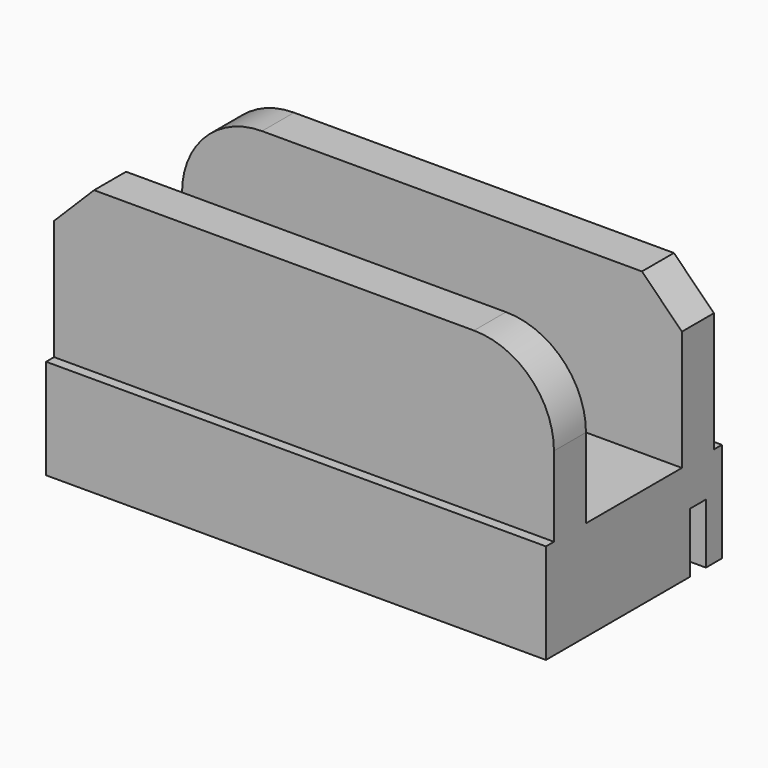
from build123d import *

# Parameters (mm, degrees)
F0_W      = 125
F0_H      = 25
F1_DEPTH  = 55
F2_W      = 125
F2_H      = 40
F3_DEPTH  = 52.5
F4_W      = 125
F4_H      = 40
F5_DEPTH  = 2.5
F6_W      = 30
F6_H      = 40
F7_DEPTH  = 125.001
F8_SIZE   = 10
F9_R      = 20
F10_SIZE  = 10
F11_R     = 20
F12_W     = 5
F12_H     = 15
F13_DEPTH = 125.001
F15_DEPTH = 25.001


with BuildPart() as f1:
    # F0 (on Front) → F1 (new body)
    with BuildSketch(Plane.XZ):
        Rectangle(F0_W, F0_H)
    extrude(amount=F1_DEPTH)

    # F2 (on face) → F3 (join)
    with BuildSketch(Plane.XZ.offset(55)):
        with Locations((0, 32.5)):
            Rectangle(F2_W, F2_H)
    extrude(amount=-F3_DEPTH)

    # F4 (on face) → F5 (cut)
    with BuildSketch(Plane.XZ.offset(55)):
        with Locations((0, 32.5)):
            Rectangle(F4_W, F4_H)
    extrude(amount=-F5_DEPTH, mode=Mode.SUBTRACT)

    # F6 (on face) → F7 (cut, through all)
    with BuildSketch(Plane(origin=(-62.5, 0, 0), x_dir=(0, -1, 0), z_dir=(-1, 0, 0))):
        with Locations((27.5, 32.5)):
            Rectangle(F6_W, F6_H)
    extrude(amount=-F7_DEPTH, mode=Mode.SUBTRACT)

    # F8
    f8_edges = [f1.edges().sort_by_distance(p)[0] for p in [
        (-62.5, -47.5, 52.5),
    ]]
    chamfer(f8_edges, length=F8_SIZE)

    # F9
    f9_edges = [f1.edges().sort_by_distance(p)[0] for p in [
        (-62.5, -7.5, 52.5),
    ]]
    fillet(f9_edges, radius=F9_R)

    # F10
    f10_edges = [f1.edges().sort_by_distance(p)[0] for p in [
        (62.5, -7.5, 52.5),
    ]]
    chamfer(f10_edges, length=F10_SIZE)

    # F11
    f11_edges = [f1.edges().sort_by_distance(p)[0] for p in [
        (62.5, -47.5, 52.5),
    ]]
    fillet(f11_edges, radius=F11_R)

    # F12 (on face) → F13 (cut, through all)
    with BuildSketch(Plane(origin=(-62.5, 0, 0), x_dir=(0, -1, 0), z_dir=(-1, 0, 0))):
        with Locations((7.5, -5)):
            Rectangle(F12_W, F12_H)
    extrude(amount=-F13_DEPTH, mode=Mode.SUBTRACT)

    # F14 (on face) → F15 (cut, through all)
    with BuildSketch(Plane.XY.offset(12.5)):
        with BuildLine():
            ThreePointArc((7e-10, -42.5), (10.606601718, -38.1066017176), (15, -27.5))
            ThreePointArc((15, -27.5), (10.6066017178, -16.8933982822), (0, -12.5))
            ThreePointArc((0, -12.5), (-15, -27.5000000003), (7e-10, -42.5))
        make_face()
    extrude(amount=-F15_DEPTH, mode=Mode.SUBTRACT)


solid = f1.part
